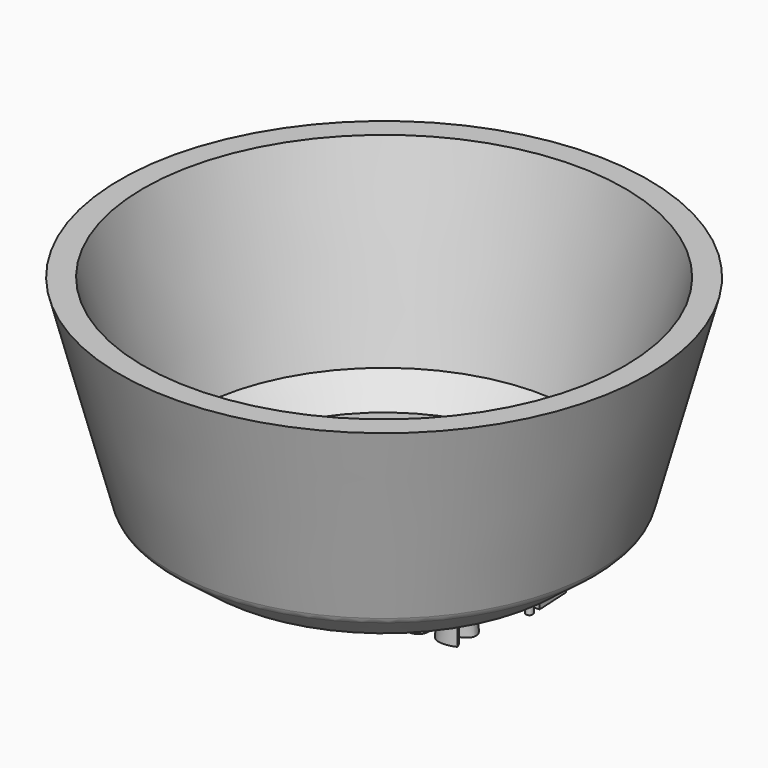
from build123d import *

# Parameters (mm, degrees)
F0_R         = 90
F1_DEPTH     = 100
F1_TAPER     = -15
F2_SIZE      = 15
F3_R         = 5
F4_T         = -10
F5_TEXT_SIZE = 29.4242551507
F6_DEPTH     = 25


# Not quite as in the source:
# - the program builds the solid bodies; features that only make, move or delete a surface that nothing else refers to are left out
# - Text() gives the source's letters only with a copy of the font that has no kerning and outlines rounded to 1/6400 em; it was checked with that copy


with BuildPart() as f1:
    # F0 (on Top) → F1 (new body)
    with BuildSketch(Plane.XY):
        Circle(F0_R)
    extrude(amount=F1_DEPTH, taper=F1_TAPER)

    # F2
    f2_edges = [f1.edges().sort_by_distance(p)[0] for p in [
        (-90, 0, 0),
    ]]
    chamfer(f2_edges, length=F2_SIZE)

    # F3
    f3_edges = [f1.edges().sort_by_distance(p)[0] for p in [
        (-93.882286, 0, 14.488887),
        (-75, 0, 0),
    ]]
    fillet(f3_edges, radius=F3_R)

    # F4
    f4_openings = [f1.faces().sort_by_distance(p)[0] for p in [
        (0, 0, 100),
    ]]
    offset(amount=F4_T, openings=f4_openings, kind=Kind.INTERSECTION)

    # F5 (on face) → F6 (join)
    with BuildSketch(Plane(origin=(0, 0, 0), x_dir=(1, 0, 0), z_dir=(0, 0, -1))):
        with Locations(Location((-50.7440801547, 2.7140363771), (0, 0, -3.0615355537))):
            Text('Raskas', F5_TEXT_SIZE, font='Open Sans', text_align=(TextAlign.LEFT, TextAlign.BOTTOM))
        with Locations(Location((-52.8813254842, -37.2458363874), (0, 0, -3.0615355537))):
            Text('Rosessi', F5_TEXT_SIZE, font='Open Sans', text_align=(TextAlign.LEFT, TextAlign.BOTTOM))
    extrude(amount=F6_DEPTH)


solid = f1.part
